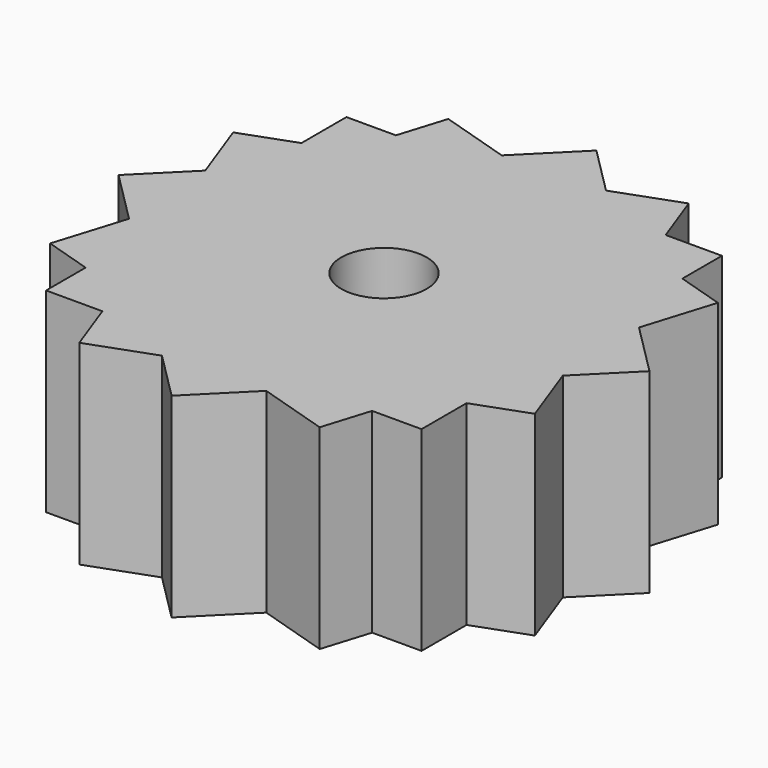
from build123d import *

# Parameters (mm, degrees)
F0_R     = 5.5579508341
F1_DEPTH = 12.7


with BuildPart() as f1:
    # F0 (on Top) → F1 (new body, symmetric)
    with BuildSketch(Plane.XY):
        with BuildLine():
            ThreePointArc((27.919055077, -5.3017102181), (28.2929762045, -2.6625673927), (28.4179831732, 0))
            ThreePointArc((28.4179831732, 0), (28.2207898632, 3.3419735383), (27.6319465947, 6.6375669502))
            ThreePointArc((27.6319465947, 6.6375669502), (27.588477608, 6.8159864218), (27.5438565796, 6.9941212708))
            ThreePointArc((27.5438565796, 6.9941212708), (20.0945486094, 20.0945486094), (6.9941212708, 27.5438565796))
            ThreePointArc((6.9941212708, 27.5438565796), (6.1507773069, 27.7443635024), (5.3017102181, 27.919055077))
            ThreePointArc((5.3017102181, 27.919055077), (2.6625673927, 28.2929762045), (0, 28.4179831732))
            ThreePointArc((0, 28.4179831732), (-3.3419735383, 28.2207898632), (-6.6375669502, 27.6319465947))
            ThreePointArc((-6.6375669502, 27.6319465947), (-6.8159864218, 27.588477608), (-6.9941212708, 27.5438565796))
            ThreePointArc((-6.9941212708, 27.5438565796), (-13.3962958665, 25.0623427613), (-19.0164091945, 21.1177164717))
            ThreePointArc((-19.0164091945, 21.1177164717), (-20.5718228566, 19.6056591827), (-22.0073683293, 17.9793633605))
            ThreePointArc((-22.0073683293, 17.9793633605), (-25.3771522917, 12.7899143545), (-27.5438565796, 6.9941212708))
            ThreePointArc((-27.5438565796, 6.9941212708), (-27.7443635024, 6.1507773069), (-27.919055077, 5.3017102181))
            ThreePointArc((-27.919055077, 5.3017102181), (-28.409770001, -0.6831808855), (-27.6319465947, -6.6375669502))
            ThreePointArc((-27.6319465947, -6.6375669502), (-27.588477608, -6.8159864218), (-27.5438565796, -6.9941212708))
            ThreePointArc((-27.5438565796, -6.9941212708), (-26.2547930089, -10.8750913416), (-24.4220383465, -14.5308571885))
            ThreePointArc((-24.4220383465, -14.5308571885), (-22.8800647164, -16.8548036537), (-21.1177164717, -19.0164091945))
            ThreePointArc((-21.1177164717, -19.0164091945), (-19.6056591827, -20.5718228566), (-17.9793633605, -22.0073683293))
            ThreePointArc((-17.9793633605, -22.0073683293), (-16.2998855168, -23.2786490109), (-14.5308571885, -24.4220383465))
            ThreePointArc((-14.5308571885, -24.4220383465), (-10.8750913416, -26.2547930089), (-6.9941212708, -27.5438565796))
            ThreePointArc((-6.9941212708, -27.5438565796), (-6.1507773069, -27.7443635024), (-5.3017102181, -27.919055077))
            ThreePointArc((-5.3017102181, -27.919055077), (-2.6625673927, -28.2929762045), (0, -28.4179831732))
            ThreePointArc((0, -28.4179831732), (3.3419735383, -28.2207898632), (6.6375669502, -27.6319465947))
            ThreePointArc((6.6375669502, -27.6319465947), (6.8159864218, -27.588477608), (6.9941212708, -27.5438565796))
            ThreePointArc((6.9941212708, -27.5438565796), (10.8750913416, -26.2547930089), (14.5308571885, -24.4220383465))
            ThreePointArc((14.5308571885, -24.4220383465), (16.8548036537, -22.8800647164), (19.0164091945, -21.1177164717))
            ThreePointArc((19.0164091945, -21.1177164717), (20.5718228566, -19.6056591827), (22.0073683293, -17.9793633605))
            ThreePointArc((22.0073683293, -17.9793633605), (23.2786490109, -16.2998855168), (24.4220383465, -14.5308571885))
            ThreePointArc((24.4220383465, -14.5308571885), (26.2547930089, -10.8750913416), (27.5438565796, -6.9941212708))
            ThreePointArc((27.5438565796, -6.9941212708), (27.7443635024, -6.1507773069), (27.919055077, -5.3017102181))
        make_face()
        Circle(F0_R, mode=Mode.SUBTRACT)
        with BuildLine():
            ThreePointArc((27.6319465947, 6.6375669502), (28.2207898632, 3.3419735383), (28.4179831732, 0))
            ThreePointArc((28.4179831732, 0), (28.2929762045, -2.6625673927), (27.919055077, -5.3017102181))
            Line((27.919055077, -5.3017102181), (28.2705482037, -6.2674296468))
            Line((28.2705482037, -6.2674296468), (34.5379778505, 0))
            Line((34.5379778505, 0), (27.6955405475, 6.8424373029))
            Line((27.6955405475, 6.8424373029), (27.6319465947, 6.6375669502))
        make_face()
        with BuildLine():
            ThreePointArc((27.5438565796, 6.9941212708), (27.588477608, 6.8159864218), (27.6319465947, 6.6375669502))
            Line((27.6319465947, 6.6375669502), (27.6955405475, 6.8424373029))
            Line((27.6955405475, 6.8424373029), (27.5438565796, 6.9941212708))
        make_face()
        with BuildLine():
            Line((28.2705482037, -6.2674296468), (27.919055077, -5.3017102181))
            ThreePointArc((27.919055077, -5.3017102181), (27.7443635024, -6.1507773069), (27.5438565796, -6.9941212708))
            Line((27.5438565796, -6.9941212708), (28.2705482037, -6.2674296468))
        make_face()
        with BuildLine():
            ThreePointArc((6.9941212708, 27.5438565796), (20.0945486094, 20.0945486094), (27.5438565796, 6.9941212708))
            Line((27.5438565796, 6.9941212708), (27.6955405475, 6.8424373029))
            Line((27.6955405475, 6.8424373029), (30.5642526553, 16.0841031339))
            Line((30.5642526553, 16.0841031339), (24.4220383465, 17.9907122754))
            Line((24.4220383465, 17.9907122754), (24.4220383465, 24.4220383465))
            Line((24.4220383465, 24.4220383465), (17.1004953487, 24.4220383465))
            Line((17.1004953487, 24.4220383465), (14.5963801632, 31.3020382744))
            Line((14.5963801632, 31.3020382744), (6.2674296468, 28.2705482037))
            Line((6.2674296468, 28.2705482037), (6.9941212708, 27.5438565796))
        make_face()
        with BuildLine():
            Line((28.2705482037, -6.2674296468), (27.5438565796, -6.9941212708))
            ThreePointArc((27.5438565796, -6.9941212708), (26.2547930089, -10.8750913416), (24.4220383465, -14.5308571885))
            Line((24.4220383465, -14.5308571885), (24.4220383465, -17.1004953487))
            Line((24.4220383465, -17.1004953487), (31.3020382744, -14.5963801632))
            Line((31.3020382744, -14.5963801632), (28.2705482037, -6.2674296468))
        make_face()
        with BuildLine():
            ThreePointArc((5.3017102181, 27.919055077), (6.1507773069, 27.7443635024), (6.9941212708, 27.5438565796))
            Line((6.9941212708, 27.5438565796), (6.2674296468, 28.2705482037))
            Line((6.2674296468, 28.2705482037), (5.3017102181, 27.919055077))
        make_face()
        with BuildLine():
            Line((24.4220383465, -17.1004953487), (24.4220383465, -14.5308571885))
            ThreePointArc((24.4220383465, -14.5308571885), (23.2786490109, -16.2998855168), (22.0073683293, -17.9793633605))
            Line((22.0073683293, -17.9793633605), (24.4220383465, -17.1004953487))
        make_face()
        with BuildLine():
            ThreePointArc((0, 28.4179831732), (2.6625673927, 28.2929762045), (5.3017102181, 27.919055077))
            Line((5.3017102181, 27.919055077), (6.2674296468, 28.2705482037))
            Line((6.2674296468, 28.2705482037), (0, 34.5379778505))
            Line((0, 34.5379778505), (-6.8424373029, 27.6955405475))
            Line((-6.8424373029, 27.6955405475), (-6.6375669502, 27.6319465947))
            ThreePointArc((-6.6375669502, 27.6319465947), (-3.3419735383, 28.2207898632), (0, 28.4179831732))
        make_face()
        with BuildLine():
            Line((24.4220383465, -17.1004953487), (22.0073683293, -17.9793633605))
            ThreePointArc((22.0073683293, -17.9793633605), (20.5718228566, -19.6056591827), (19.0164091945, -21.1177164717))
            Line((19.0164091945, -21.1177164717), (17.9907122754, -24.4220383465))
            Line((17.9907122754, -24.4220383465), (24.4220383465, -24.4220383465))
            Line((24.4220383465, -24.4220383465), (24.4220383465, -17.1004953487))
        make_face()
        with BuildLine():
            Line((17.9907122754, -24.4220383465), (19.0164091945, -21.1177164717))
            ThreePointArc((19.0164091945, -21.1177164717), (16.8548036537, -22.8800647164), (14.5308571885, -24.4220383465))
            Line((14.5308571885, -24.4220383465), (17.9907122754, -24.4220383465))
        make_face()
        with BuildLine():
            ThreePointArc((-6.9941212708, 27.5438565796), (-6.8159864218, 27.588477608), (-6.6375669502, 27.6319465947))
            Line((-6.6375669502, 27.6319465947), (-6.8424373029, 27.6955405475))
            Line((-6.8424373029, 27.6955405475), (-6.9941212708, 27.5438565796))
        make_face()
        with BuildLine():
            Line((-6.9941212708, 27.5438565796), (-6.8424373029, 27.6955405475))
            Line((-6.8424373029, 27.6955405475), (-16.0841031339, 30.5642526553))
            Line((-16.0841031339, 30.5642526553), (-17.9907122754, 24.4220383465))
            Line((-17.9907122754, 24.4220383465), (-24.4220383465, 24.4220383465))
            Line((-24.4220383465, 24.4220383465), (-24.4220383465, 17.1004953487))
            Line((-24.4220383465, 17.1004953487), (-31.3020382744, 14.5963801632))
            Line((-31.3020382744, 14.5963801632), (-28.2705482037, 6.2674296468))
            Line((-28.2705482037, 6.2674296468), (-27.5438565796, 6.9941212708))
            ThreePointArc((-27.5438565796, 6.9941212708), (-25.3771522917, 12.7899143545), (-22.0073683293, 17.9793633605))
            ThreePointArc((-22.0073683293, 17.9793633605), (-20.5718228566, 19.6056591827), (-19.0164091945, 21.1177164717))
            ThreePointArc((-19.0164091945, 21.1177164717), (-13.3962958665, 25.0623427613), (-6.9941212708, 27.5438565796))
        make_face()
        with BuildLine():
            Line((17.9907122754, -24.4220383465), (14.5308571885, -24.4220383465))
            ThreePointArc((14.5308571885, -24.4220383465), (10.8750913416, -26.2547930089), (6.9941212708, -27.5438565796))
            Line((6.9941212708, -27.5438565796), (6.8424373029, -27.6955405475))
            Line((6.8424373029, -27.6955405475), (16.0841031339, -30.5642526553))
            Line((16.0841031339, -30.5642526553), (17.9907122754, -24.4220383465))
        make_face()
        with BuildLine():
            Line((6.8424373029, -27.6955405475), (6.9941212708, -27.5438565796))
            ThreePointArc((6.9941212708, -27.5438565796), (6.8159864218, -27.588477608), (6.6375669502, -27.6319465947))
            Line((6.6375669502, -27.6319465947), (6.8424373029, -27.6955405475))
        make_face()
        with BuildLine():
            Line((6.8424373029, -27.6955405475), (6.6375669502, -27.6319465947))
            ThreePointArc((6.6375669502, -27.6319465947), (3.3419735383, -28.2207898632), (0, -28.4179831732))
            ThreePointArc((0, -28.4179831732), (-2.6625673927, -28.2929762045), (-5.3017102181, -27.919055077))
            Line((-5.3017102181, -27.919055077), (-6.2674296468, -28.2705482037))
            Line((-6.2674296468, -28.2705482037), (0, -34.5379778505))
            Line((0, -34.5379778505), (6.8424373029, -27.6955405475))
        make_face()
        with BuildLine():
            ThreePointArc((-27.919055077, 5.3017102181), (-27.7443635024, 6.1507773069), (-27.5438565796, 6.9941212708))
            Line((-27.5438565796, 6.9941212708), (-28.2705482037, 6.2674296468))
            Line((-28.2705482037, 6.2674296468), (-27.919055077, 5.3017102181))
        make_face()
        with BuildLine():
            Line((-6.2674296468, -28.2705482037), (-5.3017102181, -27.919055077))
            ThreePointArc((-5.3017102181, -27.919055077), (-6.1507773069, -27.7443635024), (-6.9941212708, -27.5438565796))
            Line((-6.9941212708, -27.5438565796), (-6.2674296468, -28.2705482037))
        make_face()
        with BuildLine():
            Line((-14.5963801632, -31.3020382744), (-6.2674296468, -28.2705482037))
            Line((-6.2674296468, -28.2705482037), (-6.9941212708, -27.5438565796))
            ThreePointArc((-6.9941212708, -27.5438565796), (-10.8750913416, -26.2547930089), (-14.5308571885, -24.4220383465))
            Line((-14.5308571885, -24.4220383465), (-17.1004953487, -24.4220383465))
            Line((-17.1004953487, -24.4220383465), (-14.5963801632, -31.3020382744))
        make_face()
        with BuildLine():
            ThreePointArc((-27.6319465947, -6.6375669502), (-28.409770001, -0.6831808855), (-27.919055077, 5.3017102181))
            Line((-27.919055077, 5.3017102181), (-28.2705482037, 6.2674296468))
            Line((-28.2705482037, 6.2674296468), (-34.5379778505, 0))
            Line((-34.5379778505, 0), (-27.6955405475, -6.8424373029))
            Line((-27.6955405475, -6.8424373029), (-27.6319465947, -6.6375669502))
        make_face()
        with BuildLine():
            ThreePointArc((-27.5438565796, -6.9941212708), (-27.588477608, -6.8159864218), (-27.6319465947, -6.6375669502))
            Line((-27.6319465947, -6.6375669502), (-27.6955405475, -6.8424373029))
            Line((-27.6955405475, -6.8424373029), (-27.5438565796, -6.9941212708))
        make_face()
        with BuildLine():
            Line((-17.1004953487, -24.4220383465), (-14.5308571885, -24.4220383465))
            ThreePointArc((-14.5308571885, -24.4220383465), (-16.2998855168, -23.2786490109), (-17.9793633605, -22.0073683293))
            Line((-17.9793633605, -22.0073683293), (-17.1004953487, -24.4220383465))
        make_face()
        with BuildLine():
            Line((-24.4220383465, -24.4220383465), (-17.1004953487, -24.4220383465))
            Line((-17.1004953487, -24.4220383465), (-17.9793633605, -22.0073683293))
            ThreePointArc((-17.9793633605, -22.0073683293), (-19.6056591827, -20.5718228566), (-21.1177164717, -19.0164091945))
            Line((-21.1177164717, -19.0164091945), (-24.4220383465, -17.9907122754))
            Line((-24.4220383465, -17.9907122754), (-24.4220383465, -24.4220383465))
        make_face()
        with BuildLine():
            ThreePointArc((-24.4220383465, -14.5308571885), (-26.2547930089, -10.8750913416), (-27.5438565796, -6.9941212708))
            Line((-27.5438565796, -6.9941212708), (-27.6955405475, -6.8424373029))
            Line((-27.6955405475, -6.8424373029), (-30.5642526553, -16.0841031339))
            Line((-30.5642526553, -16.0841031339), (-24.4220383465, -17.9907122754))
            Line((-24.4220383465, -17.9907122754), (-24.4220383465, -14.5308571885))
        make_face()
        with BuildLine():
            ThreePointArc((-21.1177164717, -19.0164091945), (-22.8800647164, -16.8548036537), (-24.4220383465, -14.5308571885))
            Line((-24.4220383465, -14.5308571885), (-24.4220383465, -17.9907122754))
            Line((-24.4220383465, -17.9907122754), (-21.1177164717, -19.0164091945))
        make_face()
    extrude(amount=F1_DEPTH, both=True)


solid = f1.part
